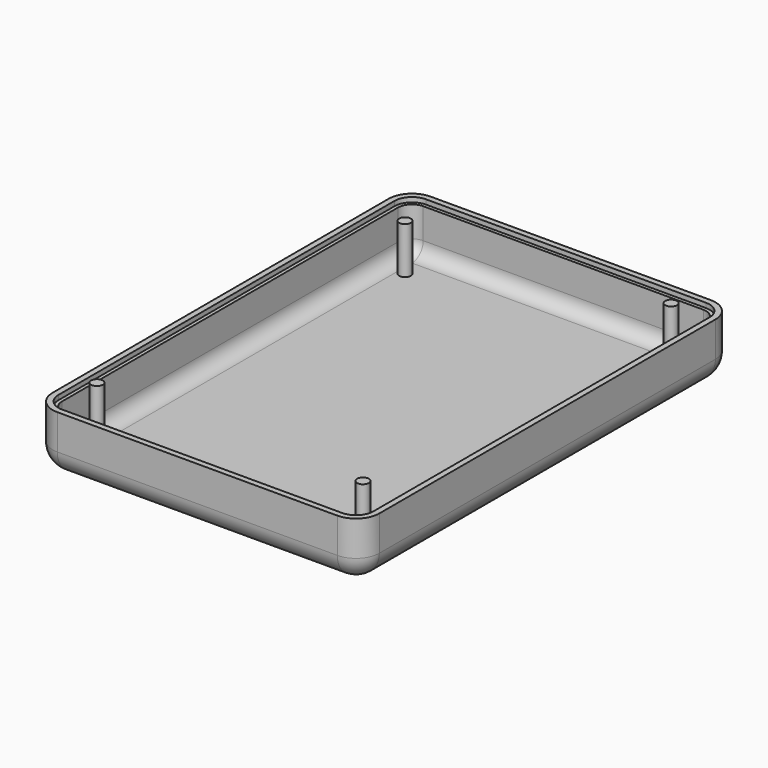
from build123d import *

# Parameters (mm, degrees)
F0_W     = 140
F0_H     = 200
F1_DEPTH = 25
F2_R     = 10
F3_T     = -4
F5_DEPTH = 2
F6_R     = 2.5
F7_DEPTH = 26
F8_R     = 2.5
F9_DEPTH = 6


with BuildPart() as f1:
    # F0 (on Top) → F1 (new body)
    with BuildSketch(Plane.XY):
        with Locations((-70, 100)):
            Rectangle(F0_W, F0_H)
    extrude(amount=F1_DEPTH)

    # F2
    f2_edges = [f1.edges().sort_by_distance(p)[0] for p in [
        (-70, 0, 0),
        (-140, 100, 0),
        (-70, 200, 0),
        (0, 100, 0),
        (-140, 0, 12.5),
        (0, 0, 12.5),
        (0, 200, 12.5),
        (-140, 200, 12.5),
    ]]
    fillet(f2_edges, radius=F2_R)

    # F3
    f3_openings = [f1.faces().sort_by_distance(p)[0] for p in [
        (-70, 100, 25),
    ]]
    offset(amount=F3_T, openings=f3_openings)

    # F4 (on face) → F5 (cut)
    with BuildSketch(Plane.XY.offset(25)):
        with BuildLine():
            Line((-2.5, 10), (-2.5, 190))
            ThreePointArc((-2.5, 190), (-4.6966991411, 195.3033008589), (-10, 197.5))
            Line((-10, 197.5), (-130, 197.5))
            ThreePointArc((-130, 197.5), (-135.3033008589, 195.3033008589), (-137.5, 190))
            Line((-137.5, 190), (-137.5, 10))
            ThreePointArc((-137.5, 10), (-135.3033008589, 4.6966991411), (-130, 2.5))
            Line((-130, 2.5), (-10, 2.5))
            ThreePointArc((-10, 2.5), (-4.6966991411, 4.6966991411), (-2.5, 10))
        make_face()
        with BuildLine():
            ThreePointArc((-136, 190), (-134.2426406871, 194.2426406871), (-130, 196))
            Line((-130, 196), (-10, 196))
            ThreePointArc((-10, 196), (-5.7573593129, 194.2426406871), (-4, 190))
            Line((-4, 190), (-4, 10))
            ThreePointArc((-4, 10), (-5.7573593129, 5.7573593129), (-10, 4))
            Line((-10, 4), (-130, 4))
            ThreePointArc((-130, 4), (-134.2426406871, 5.7573593129), (-136, 10))
            Line((-136, 10), (-136, 190))
        make_face(mode=Mode.SUBTRACT)
    extrude(amount=-F5_DEPTH, mode=Mode.SUBTRACT)

    # F6 (on face) → F7 (join)
    with BuildSketch(Plane.XY.offset(4)):
        with Locations((-127, 182.5)):
            Circle(F6_R)
        with Locations((-13, 182.5)):
            Circle(F6_R)
        with Locations((-127, 17.5)):
            Circle(F6_R)
        with Locations((-13, 17.5)):
            Circle(F6_R)
    extrude(amount=F7_DEPTH)

    # F8 (on face) → F9 (cut)
    with BuildSketch(Plane.XY.offset(30)):
        with Locations((-127, 182.5)):
            Circle(F8_R)
    extrude(amount=-F9_DEPTH, mode=Mode.SUBTRACT)


solid = f1.part
